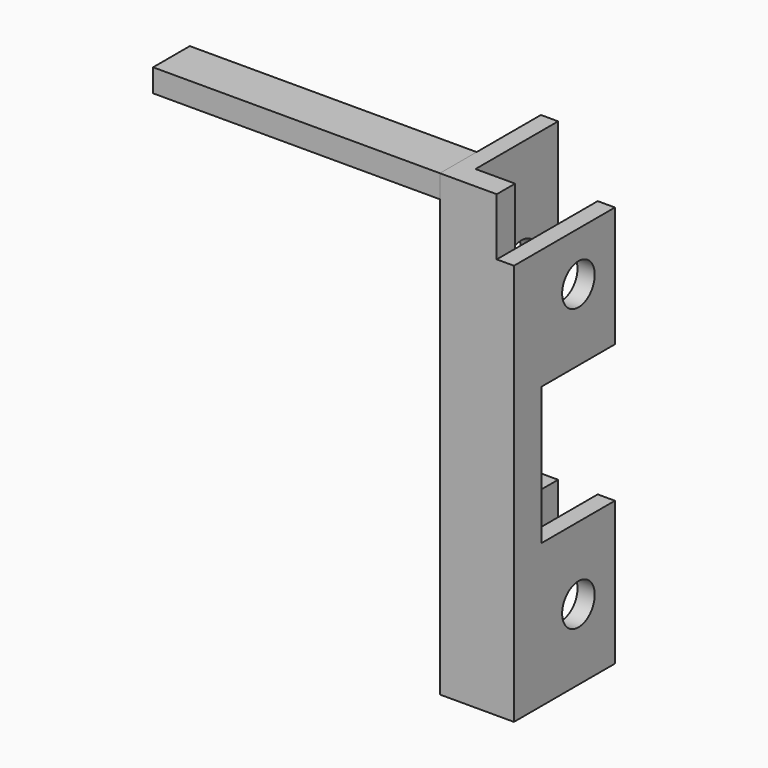
from build123d import *

# Parameters (mm, degrees)
F1_DEPTH = 70
F2_R     = 3.55
F3_DEPTH = 12.901
F5_DEPTH = 10
F6_W     = 8
F6_H     = 4
F7_DEPTH = 50
F8_W     = 9.9
F8_H     = 24
F8_W_2   = 3
F9_DEPTH = 16


# Not quite as in the source:
# - a feature names something its author has since deleted; it is built from what else it names


with BuildPart() as f1:
    # F0 (on Top) → F1 (new body)
    with BuildSketch(Plane.XY):
        Polygon((0, 22), (0, 0), (12.9, 0), (12.9, 22), (9.9, 22), (9.9, 4), (3, 4), (3, 22), align=None)
    extrude(amount=F1_DEPTH)

    # F2 (on face) → F3 (cut, through all)
    with BuildSketch(Plane.YZ.offset(12.9)):
        with Locations((14.05, 61.45)):
            Circle(F2_R)
        with Locations((14.05, 12.35)):
            Circle(F2_R)
    extrude(amount=-F3_DEPTH, mode=Mode.SUBTRACT)

    # F4 (on face) → F5 (join)
    with BuildSketch(Plane.XY.offset(70)):
        Polygon((9.9, 0), (9.9, 4), (3, 4), (3, 22), (0, 22), (0, 0), align=None)
    extrude(amount=F5_DEPTH)

    # F8 (on face) → F9 (cut)
    with BuildSketch(Plane(origin=(0, 22, 0), x_dir=(-1, 0, 0), z_dir=(0, 1, 0))):
        with Locations((-4.95, 37)):
            Rectangle(F8_W, F8_H)
        with Locations((-11.4, 37)):
            Rectangle(F8_W_2, F8_H)
    extrude(amount=-F9_DEPTH, mode=Mode.SUBTRACT)


with BuildPart() as f7:
    # F6 (on face) → F7 (new body)
    with BuildSketch(Plane(origin=(0, 0, 0), x_dir=(0, -1, 0), z_dir=(-1, 0, 0))):
        with Locations((-4, 78)):
            Rectangle(F6_W, F6_H)
    extrude(amount=F7_DEPTH)


solid = Compound([f1.part, f7.part])
